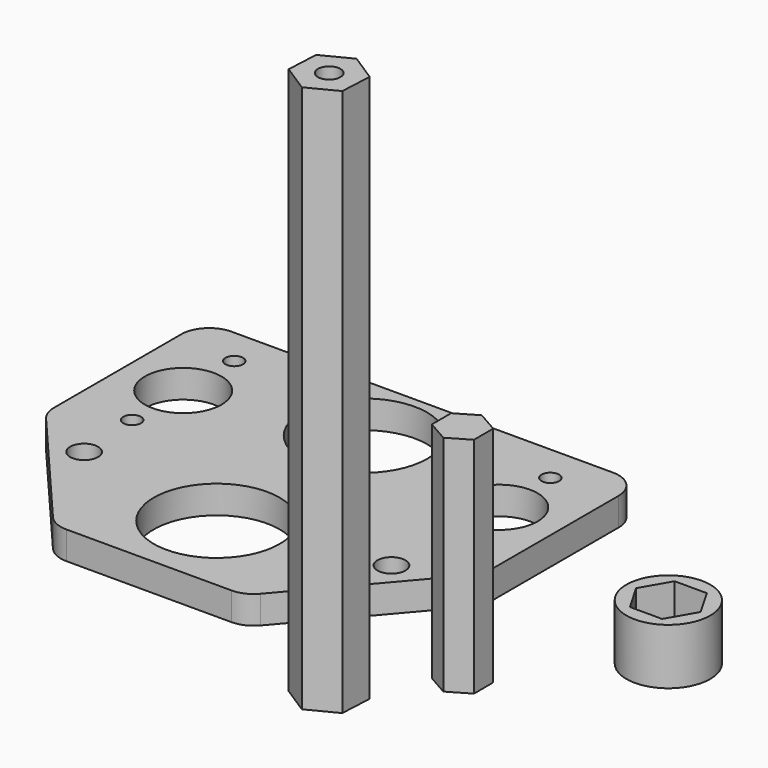
from build123d import *

# Parameters (mm, degrees)
F0_R     = 14.2875
F0_R_2   = 3.175
F0_R_3   = 2
F0_R_4   = 8.6995
F1_DEPTH = 6.35
F2_R     = 6.35
F4_DEPTH = 50.8
F5_R     = 2.5527
F6_DEPTH = 124.46
F7_R     = 9.525
F8_DEPTH = 12.7


# Not quite as in the source:
# - a length typed as a fraction of an inch, garbled in the dataset ("3 / 203.2 mm" for 3/8 in), is restored


with BuildPart() as f1:
    # F0 (on Top) → F1 (new body)
    with BuildSketch(Plane.XY):
        Polygon((-3.3328348122, 43.7322813914), (-102.7379401762, 43.7322813914), (-102.7379401762, -1.147727031), (-74.7225361252, -33.9411287354), (-31.3482388633, -33.9411287354), (-3.3328348122, -1.147727031), align=None)
        with Locations((-53.0353874942, -14.6743590031)):
            Circle(F0_R, mode=Mode.SUBTRACT)
        with Locations((-87.9603874942, -8.6888484657)):
            Circle(F0_R_2, mode=Mode.SUBTRACT)
        with Locations((-18.1103874942, -8.6888484657)):
            Circle(F0_R_2, mode=Mode.SUBTRACT)
        with Locations((-88.9584401762, 6.1979512684)):
            Circle(F0_R_3, mode=Mode.SUBTRACT)
        with Locations((-88.9584401762, 20.7013512684)):
            Circle(F0_R_4, mode=Mode.SUBTRACT)
        with Locations((-88.9584401762, 35.2047512684)):
            Circle(F0_R_3, mode=Mode.SUBTRACT)
        with Locations((-53.0353874942, 27.2356409969)):
            Circle(F0_R, mode=Mode.SUBTRACT)
        with Locations((-17.1123348122, 6.1979512684)):
            Circle(F0_R_3, mode=Mode.SUBTRACT)
        with Locations((-17.1123348122, 20.7013512684)):
            Circle(F0_R_4, mode=Mode.SUBTRACT)
        with Locations((-17.1123348122, 35.2047512684)):
            Circle(F0_R_3, mode=Mode.SUBTRACT)
    extrude(amount=F1_DEPTH)

    # F2
    f2_edges = [f1.edges().sort_by_distance(p)[0] for p in [
        (-102.73794, 43.732281, 3.175),
        (-102.73794, -1.147727, 3.175),
        (-74.722536, -33.941129, 3.175),
        (-31.348239, -33.941129, 3.175),
        (-3.332835, -1.147727, 3.175),
        (-3.332835, 43.732281, 3.175),
    ]]
    fillet(f2_edges, radius=F2_R)


with BuildPart() as f4:
    # F3 (on Top) → F4 (new body)
    with BuildSketch(Plane.XY):
        Polygon((11.7561597103, -31.2877350769), (16.5063053389, -28.5168161847), (16.4816920008, -23.0176099525), (11.706933034, -20.2893226126), (6.9567874054, -23.0602415048), (6.9814007436, -28.5594477369), align=None)
    extrude(amount=F4_DEPTH)


with BuildPart() as f6:
    # F5 (on Top) → F6 (new body)
    with BuildSketch(Plane.XY):
        Polygon((-3.6010059256, -52.2956447094), (2.9234465559, -48.9497736496), (3.2880634611, -41.6264965249), (-2.8717721153, -37.64909046), (-9.3962245969, -40.9949615198), (-9.760841502, -48.3182386445), align=None)
        with Locations((-3.2363890205, -44.9723675847)):
            Circle(F5_R, mode=Mode.SUBTRACT)
    extrude(amount=F6_DEPTH)


with BuildPart() as f8:
    # F7 (on Top) → F8 (new body)
    with BuildSketch(Plane.XY):
        with Locations((36.2145788968, 2.0721156616)):
            Circle(F7_R)
        Polygon((43.5469273155, 2.0721156616), (39.8807531061, -4.2778843384), (32.5484046874, -4.2778843384), (28.8822304781, 2.0721156616), (32.5484046874, 8.4221156616), (39.8807531061, 8.4221156616), align=None, mode=Mode.SUBTRACT)
    extrude(amount=F8_DEPTH)


solid = Compound([f1.part, f4.part, f6.part, f8.part])
